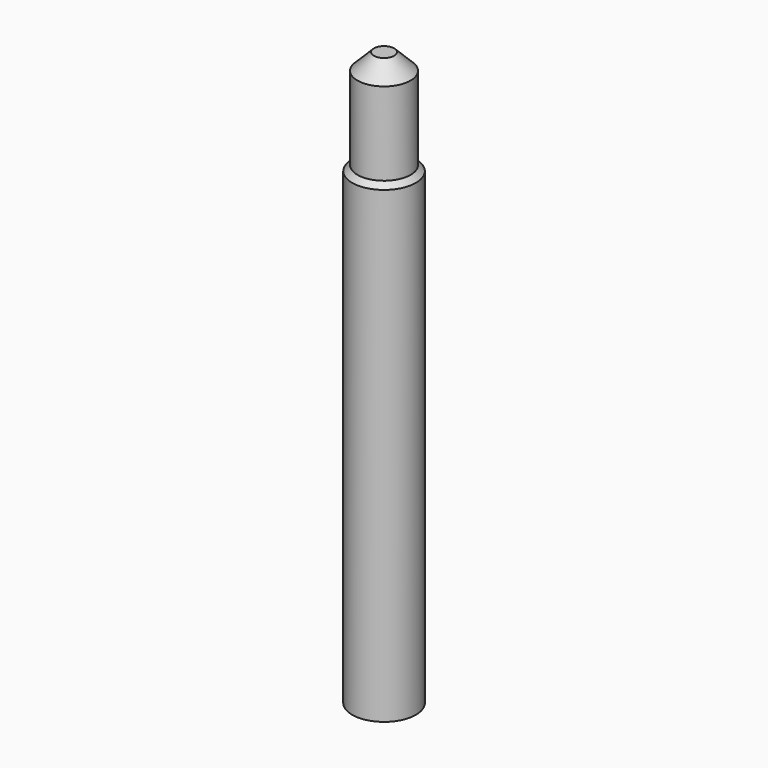
from build123d import *

# Parameters (mm, degrees)
F0_R        = 9.8428256451
F0_R_2      = 8.2055899986
F1_DEPTH    = 25.4
F2_DEPTH    = 115.824
F3_DEPTH    = 61.214
F3_FACE_R   = 8.2055899986
F6_S5_R     = 9.8428256451
F6_T6_DEPTH = 20
F5_R        = 7.5988621304
F7_DEPTH    = 107.188
F8_W        = 0.8552042418
F8_H        = 3.9967889898
F8_W_2      = 3.9967889898
F8_H_2      = 0.8552042418
F9_DEPTH    = 6.35


# Not quite as in the source:
# - a fillet or chamfer that OpenCascade refuses, or shapes differently, is made with other operations: its cross-section is extruded or revolved along the edge and cut away or added


with BuildPart() as f1:
    # F0 (on Top) → F1 (new body)
    with BuildSketch(Plane.XY):
        Circle(F0_R)
        Circle(F0_R_2, mode=Mode.SUBTRACT)
    extrude(amount=F1_DEPTH)

    # F2 (add): a face of the model
    f2_faces = [f1.faces().sort_by_distance(p)[0] for p in [
        (-9.5644284947, 0, 0),
    ]]
    extrude(f2_faces, amount=F2_DEPTH)

    # F0 (on Top) → F3 (join)
    with BuildSketch(Plane.XY):
        Circle(F0_R_2)
    extrude(amount=F3_DEPTH)

    # F3_face (on face) → F4 section 0
    with BuildSketch(Plane.XY.offset(61.214), mode=Mode.PRIVATE) as f4_s0:
        Circle(F3_FACE_R)
    loft([Vertex(0, 0, 0), f4_s0.sketch])

    # F6: chamfer of 5.08 on 3 edges, made by hand


with BuildPart() as f6_tool2:
    # F6_s3 → F6_t4 (revolve)
    with BuildSketch(Plane.XZ):
        Polygon((13.2855899986, 25.4), (8.2055899986, 30.48), (8.2055899986, 25.4), align=None)
    revolve(axis=Axis((0, 0, 25.4), (0, 0, 1)))

    # F6_s5 → F6_t6 (intersect, symmetric)
    with BuildSketch(Plane.XY.offset(27.9)):
        Circle(F6_S5_R)
    extrude(amount=F6_T6_DEPTH, both=True, mode=Mode.INTERSECT)


with BuildPart() as f1_1:
    add(f1.part)

    # F6_t1: union F6_tool2
    add(f6_tool2.part)

    # F6_s7 → F6_t8 (revolve, cut)
    with BuildSketch(Plane.XZ):
        Polygon((8.2055899986, 56.134), (3.1255899986, 61.214), (8.2055899986, 61.214), align=None)
    revolve(axis=Axis((0, 0, 61.214), (0, 0, 1)), mode=Mode.SUBTRACT)

    # F5 (on Top) → F7 (join)
    with BuildSketch(Plane.XY):
        Circle(F5_R)
    extrude(amount=-F7_DEPTH)

    # F8 (on face) → F9 (join)
    with BuildSketch(Plane(origin=(0, 0, -107.188), x_dir=(1, 0, 0), z_dir=(0, 0, -1))):
        with Locations((0.0061568862, 6.3575312961)):
            Rectangle(F8_W, F8_H)
        Polygon((-6.2065385732, 5.6105250065), (-3.3803819756, 2.7843684089), (-2.7756612569, 3.3890891276), (-5.6018178545, 6.2152457252), align=None)
        with Locations((-6.3575312961, 0.0061568862)):
            Rectangle(F8_W_2, F8_H_2)
        Polygon((-5.6105250065, -6.2065385732), (-2.7843684089, -3.3803819756), (-3.3890891276, -2.7756612569), (-6.2152457252, -5.6018178545), align=None)
        with Locations((-0.0061568862, -6.3575312961)):
            Rectangle(F8_W, F8_H)
        Polygon((6.2065385732, -5.6105250065), (3.3803819756, -2.7843684089), (2.7756612569, -3.3890891276), (5.6018178545, -6.2152457252), align=None)
        with Locations((6.3575312961, -0.0061568862)):
            Rectangle(F8_W_2, F8_H_2)
        Polygon((5.6105250065, 6.2065385732), (2.7843684089, 3.3803819756), (3.3890891276, 2.7756612569), (6.2152457252, 5.6018178545), align=None)
    extrude(amount=F9_DEPTH)


solid = f1_1.part
